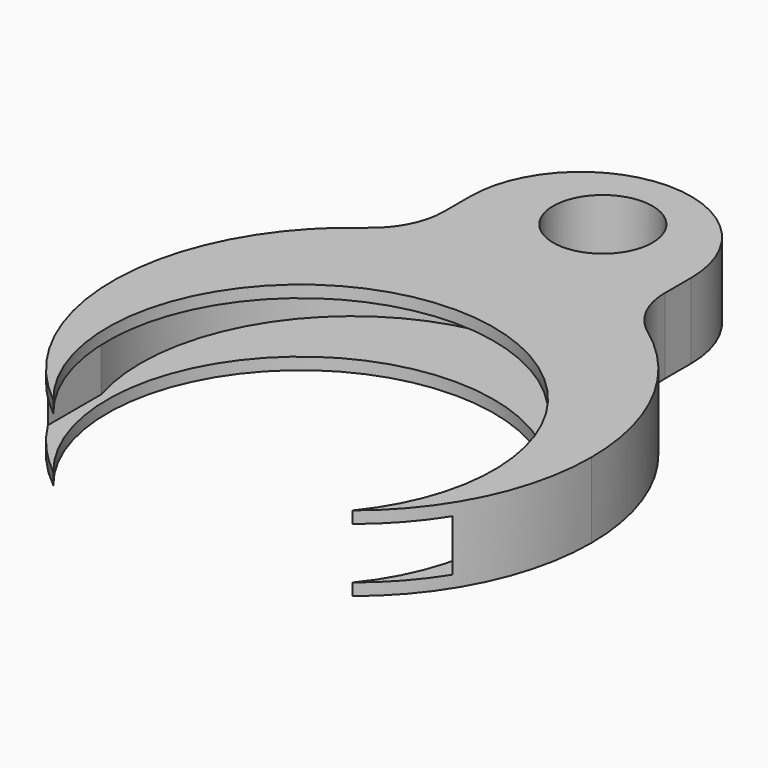
from build123d import *

# Parameters (mm, degrees)
F0_R     = 2.7
F1_DEPTH = 2.05
F2_R     = 5.99999
F3_R     = 4
F4_R     = 10.5
F5_DEPTH = 4.101
F7_DEPTH = 1.4


# Not quite as in the source:
# - a fillet or chamfer is up to 0.001 mm smaller than in the source, because OpenCascade refuses the exact size


with BuildPart() as f1:
    # F0 (on Top) → F1 (new body, symmetric)
    with BuildSketch(Plane.XY):
        with BuildLine():
            ThreePointArc((-6, 11.5325625947), (-6.7453687816, -11.1130553854), (13, 0))
            ThreePointArc((13, 0), (11.1130553854, 6.7453687816), (6, 11.5325625947))
            Line((6, 11.5325625947), (-6, 11.5325625947))
        make_face()
        with BuildLine():
            Line((-6, 11.5325625947), (6, 11.5325625947))
            ThreePointArc((6, 11.5325625947), (0, 13), (-6, 11.5325625947))
        make_face()
        with BuildLine():
            ThreePointArc((-6, 11.5325625947), (0, 13), (6, 11.5325625947))
            Line((6, 11.5325625947), (6, 21.5325625947))
            Line((6, 21.5325625947), (-6, 21.5325625947))
            Line((-6, 21.5325625947), (-6, 11.5325625947))
        make_face()
        with Locations((0, 17.0325625947)):
            Circle(F0_R, mode=Mode.SUBTRACT)
    extrude(amount=F1_DEPTH, both=True)

    # F2 (radius 6 in the source; OpenCascade refuses exactly that, so slightly less here)
    f2_edges = [f1.edges().sort_by_distance(p)[0] for p in [
        (-6, 21.532563, 0),
        (6, 21.532563, 0),
    ]]
    fillet(f2_edges, radius=F2_R)

    # F3
    f3_edges = [f1.edges().sort_by_distance(p)[0] for p in [
        (6, 11.532563, 0),
        (-6, 11.532563, 0),
    ]]
    fillet(f3_edges, radius=F3_R)

    # F4 (on face) → F5 (cut, through all)
    with BuildSketch(Plane.XY.offset(2.05)):
        with Locations((0, -3.5)):
            Circle(F4_R)
    extrude(amount=-F5_DEPTH, mode=Mode.SUBTRACT)

    # F6 (on Top) → F7 (cut, symmetric)
    with BuildSketch(Plane.XY):
        with BuildLine():
            ThreePointArc((11, -3.3115318698), (11.3650882253, -1.6736227042), (11.4876561284, 0))
            ThreePointArc((11.4876561284, 0), (-1.6736227042, 11.3650882253), (-11, -3.3115318698))
            Line((-11, -3.3115318698), (11, -3.3115318698))
        make_face()
        with BuildLine():
            Line((11, -3.3115318698), (-11, -3.3115318698))
            ThreePointArc((-11, -3.3115318698), (0, -11.4876561284), (11, -3.3115318698))
        make_face()
        with BuildLine():
            ThreePointArc((11, -3.3115318698), (0, -11.4876561284), (-11, -3.3115318698))
            Line((-11, -3.3115318698), (-11, -30.7711608721))
            Line((-11, -30.7711608721), (11, -30.7711608721))
            Line((11, -30.7711608721), (11, -3.3115318698))
        make_face()
    extrude(amount=F7_DEPTH, both=True, mode=Mode.SUBTRACT)


solid = f1.part
